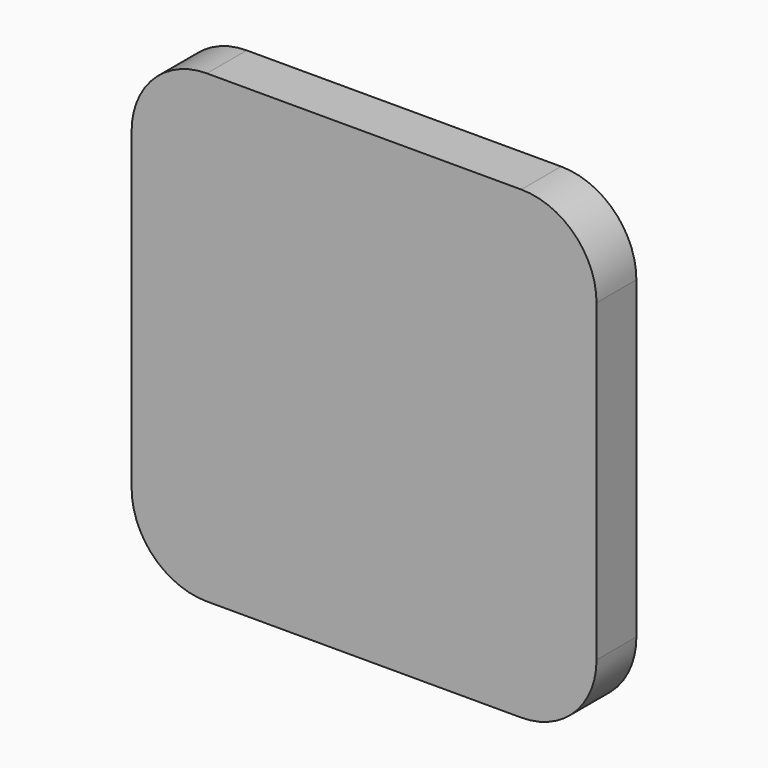
from build123d import *

# Parameters (mm, degrees)
F1_DEPTH = 19.05


# Not quite as in the source:
# - a feature names something its author has since deleted; it is built from what else it names


with BuildPart() as f1:
    # F0 (on Front) → F1 (new body)
    with BuildSketch(Plane.XZ):
        with BuildLine():
            ThreePointArc((0, 28.7803760395), (8.4295769769, 8.4295769769), (28.7803760395, 0))
            Line((28.7803760395, 0), (149.0196239605, 0))
            ThreePointArc((149.0196239605, 0), (169.3704230231, 8.4295769769), (177.8, 28.7803760395))
            Line((177.8, 28.7803760395), (177.8, 149.0196239605))
            ThreePointArc((177.8, 149.0196239605), (169.3704230231, 169.3704230231), (149.0196239605, 177.8))
            Line((149.0196239605, 177.8), (28.7803760395, 177.8))
            ThreePointArc((28.7803760395, 177.8), (8.4295769769, 169.3704230231), (0, 149.0196239605))
            Line((0, 149.0196239605), (0, 28.7803760395))
        make_face()
    extrude(amount=F1_DEPTH)


solid = f1.part
